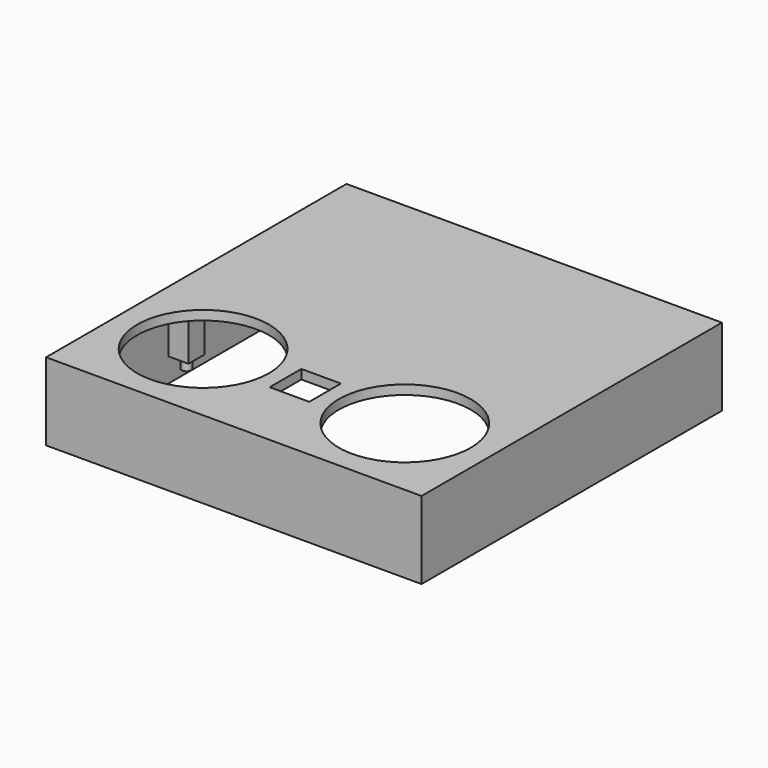
from build123d import *

# Parameters (mm, degrees)
F0_W     = 23
F0_H     = 23
F0_R     = 8.5
F1_DEPTH = 0.6
F3_DEPTH = 10
F4_W     = 2.6
F4_H     = 2.6
F4_R     = 0.6
F5_DEPTH = 5.7
F6_DEPTH = 7.2


with BuildPart() as f1:
    # F0 (on Top) → F1 (new body, symmetric)
    with BuildSketch(Plane.XY):
        with Locations((-11.5, 11.5)):
            Rectangle(F0_W, F0_H)
        Polygon((0, -10.1312079445), (0, 0), (-23, 0), (-23, -23), (0, -23), (0, -15.2312079445), (-2.55, -15.2312079445), (-2.55, -10.1312079445), align=None)
        with Locations((-13, -12.9)):
            Circle(F0_R, mode=Mode.SUBTRACT)
        with Locations((11.5, 11.5)):
            Rectangle(F0_W, F0_H)
        Polygon((23, 0), (0, 0), (0, -10.1312079445), (2.55, -10.1312079445), (2.55, -15.2312079445), (0, -15.2312079445), (0, -23), (23, -23), align=None)
        with Locations((13, -12.9)):
            Circle(F0_R, mode=Mode.SUBTRACT)
    extrude(amount=F1_DEPTH, both=True)

    # F2 (on face) → F3 (join)
    with BuildSketch(Plane.XY.offset(0.6)):
        Polygon((0, 23), (23, 23), (23, -23), (0, -23), (0, -24.2), (24.2, -24.2), (24.2, 24.2), (0, 24.2), align=None)
        Polygon((-23, 23), (0, 23), (0, 24.2), (-24.2, 24.2), (-24.2, -24.2), (0, -24.2), (0, -23), (-23, -23), align=None)
    extrude(amount=-F3_DEPTH)

    # F4 (on face) → F5 (join)
    with BuildSketch(Plane(origin=(0, 0, -0.6), x_dir=(1, 0, 0), z_dir=(0, 0, -1))):
        with Locations((21.7, 21.7)):
            Rectangle(F4_W, F4_H)
        with Locations((21.7, 21.7)):
            Circle(F4_R, mode=Mode.SUBTRACT)
        with Locations((-21.7, 21.7)):
            Rectangle(F4_W, F4_H)
        with Locations((-21.7, 21.7)):
            Circle(F4_R, mode=Mode.SUBTRACT)
        with Locations((-21.7, 4.7)):
            Rectangle(F4_W, F4_H)
        with Locations((-21.7, 4.7)):
            Circle(F4_R, mode=Mode.SUBTRACT)
        with Locations((21.7, 4.7000000451)):
            Rectangle(F4_W, F4_H)
        with Locations((21.7, 4.7000000451)):
            Circle(F4_R, mode=Mode.SUBTRACT)
    extrude(amount=F5_DEPTH)

    # F6 (add): faces of the model
    f6_faces = [f1.faces().sort_by_distance(p)[0] for p in [
        (-21.7, -4.7, -0.6),
        (-21.7, -21.7, -0.6),
        (21.7, -21.7, -0.6),
        (21.7, -4.7000000451, -0.6),
    ]]
    extrude(f6_faces, amount=F6_DEPTH)


solid = f1.part
